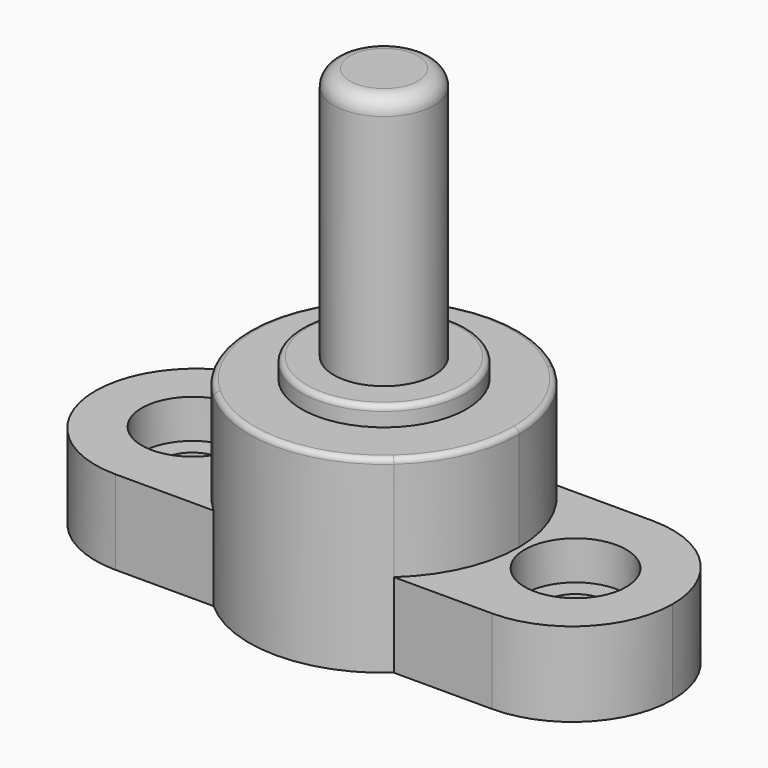
from build123d import *
from build123d import SkipClean  # not in build123d's __all__

# Parameters (mm, degrees)
F0_R           = 7.65
F0_R_2         = 4.65
F1_DEPTH       = 7.8
F2_DEPTH       = 9.7
F3_DEPTH       = 11.5
F4_DEPTH       = 35
F5_D           = 5.75
F5_CBORE_D     = 9.4
F5_CBORE_DEPTH = 3.6
F6_R           = 0.5
F7_R           = 1.5


# Not quite as in the source:
# - after a boolean that leaves OpenCascade's solid faulty, fix() repairs it


with BuildPart() as f1:
    # F0 (on Top) → F1 (new body)
    with BuildSketch(Plane.XY):
        with BuildLine():
            ThreePointArc((-8.3522452071, -9.3), (-12.5, 0), (-8.3522452071, 9.3))
            Line((-8.3522452071, 9.3), (-17.45, 9.3))
            ThreePointArc((-17.45, 9.3), (-24.026093065, 6.576093065), (-26.75, 0))
            ThreePointArc((-26.75, 0), (-24.026093065, -6.576093065), (-17.45, -9.3))
            Line((-17.45, -9.3), (-8.3522452071, -9.3))
        make_face()
        with BuildLine():
            ThreePointArc((12.5, 0), (11.4160646698, 5.0915093494), (8.3522452071, 9.3))
            Line((8.3522452071, 9.3), (-8.3522452071, 9.3))
            ThreePointArc((-8.3522452071, 9.3), (-12.5, 0), (-8.3522452071, -9.3))
            Line((-8.3522452071, -9.3), (8.3522452071, -9.3))
            ThreePointArc((8.3522452071, -9.3), (11.4160646698, -5.0915093494), (12.5, 0))
        make_face()
        Circle(F0_R, mode=Mode.SUBTRACT)
        Circle(F0_R)
        Circle(F0_R_2, mode=Mode.SUBTRACT)
        Circle(F0_R_2)
        with BuildLine():
            ThreePointArc((26.75, 0), (24.026093065, 6.576093065), (17.45, 9.3))
            Line((17.45, 9.3), (8.3522452071, 9.3))
            ThreePointArc((8.3522452071, 9.3), (11.4160646698, 5.0915093494), (12.5, 0))
            ThreePointArc((12.5, 0), (11.4160646698, -5.0915093494), (8.3522452071, -9.3))
            Line((8.3522452071, -9.3), (17.45, -9.3))
            ThreePointArc((17.45, -9.3), (24.026093065, -6.576093065), (26.75, 0))
        make_face()
        with BuildLine():
            Line((-8.3522452071, 9.3), (8.3522452071, 9.3))
            ThreePointArc((8.3522452071, 9.3), (0, 12.5), (-8.3522452071, 9.3))
        make_face()
        with BuildLine():
            ThreePointArc((-8.3522452071, -9.3), (0, -12.5), (8.3522452071, -9.3))
            Line((8.3522452071, -9.3), (-8.3522452071, -9.3))
        make_face()
    extrude(amount=-F1_DEPTH)

    # F0 (on Top) → F2 (join)
    with BuildSketch(Plane.XY):
        with BuildLine():
            Line((-8.3522452071, 9.3), (8.3522452071, 9.3))
            ThreePointArc((8.3522452071, 9.3), (0, 12.5), (-8.3522452071, 9.3))
        make_face()
        with BuildLine():
            ThreePointArc((-8.3522452071, -9.3), (0, -12.5), (8.3522452071, -9.3))
            Line((8.3522452071, -9.3), (-8.3522452071, -9.3))
        make_face()
        with BuildLine():
            ThreePointArc((12.5, 0), (11.4160646698, 5.0915093494), (8.3522452071, 9.3))
            Line((8.3522452071, 9.3), (-8.3522452071, 9.3))
            ThreePointArc((-8.3522452071, 9.3), (-12.5, 0), (-8.3522452071, -9.3))
            Line((-8.3522452071, -9.3), (8.3522452071, -9.3))
            ThreePointArc((8.3522452071, -9.3), (11.4160646698, -5.0915093494), (12.5, 0))
        make_face()
        Circle(F0_R, mode=Mode.SUBTRACT)
        Circle(F0_R)
        Circle(F0_R_2, mode=Mode.SUBTRACT)
        Circle(F0_R_2)
    with SkipClean():  # cleaning this boolean's faces spoils the solid; the shape is the same uncleaned
        extrude(amount=F2_DEPTH)

    # F0 (on Top) → F3 (join)
    with BuildSketch(Plane.XY):
        Circle(F0_R)
        Circle(F0_R_2, mode=Mode.SUBTRACT)
        Circle(F0_R_2)
    extrude(amount=F3_DEPTH)

    add(f1.part.fix(), mode=Mode.REPLACE)

    # F0 (on Top) → F4 (join)
    with BuildSketch(Plane.XY):
        Circle(F0_R_2)
    extrude(amount=F4_DEPTH)

    # F5 (through all)
    with Locations(Plane.XY):
        with Locations((-17.75, 0), (17.75, 0)):
            CounterBoreHole(F5_D / 2, F5_CBORE_D / 2, F5_CBORE_DEPTH)

    # F6
    f6_edges = [f1.edges().sort_by_distance(p)[0] for p in [
        (8.352245, -9.3, 9.7),
        (-7.65, 0, 11.5),
    ]]
    fillet(f6_edges, radius=F6_R)

    # F7
    f7_edges = [f1.edges().sort_by_distance(p)[0] for p in [
        (-4.65, 0, 35),
    ]]
    fillet(f7_edges, radius=F7_R)


solid = f1.part
